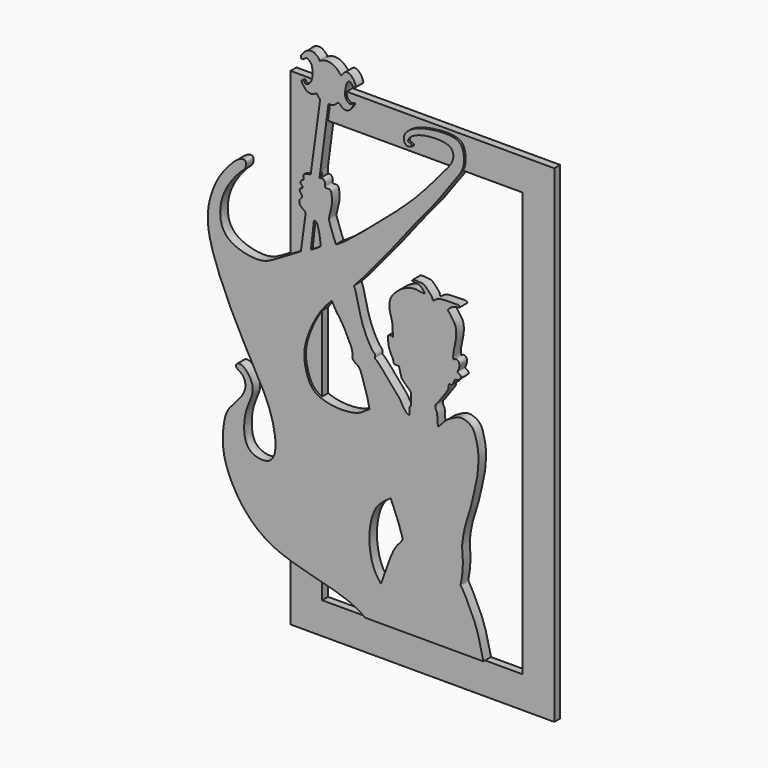
from build123d import *

# Parameters (mm, degrees)
F0_W     = 63.5
F0_H     = 117.348
F0_W_2   = 48.26
F0_H_2   = 102.108
F1_DEPTH = 1.778
F3_DEPTH = 2.286


# Not quite as in the source:
# - the program builds the solid bodies; features that only make, move or delete a surface that nothing else refers to are left out


with BuildPart() as f1:
    # F0 (on Front) → F1 (new body)
    with BuildSketch(Plane.XZ):
        Rectangle(F0_W, F0_H)
        Rectangle(F0_W_2, F0_H_2, mode=Mode.SUBTRACT)
    extrude(amount=F1_DEPTH)

    # F2 (on Front) → F3 (join)
    with BuildSketch(Plane.XZ):
        with BuildLine():
            add(Edge.make_bspline(
                [(-28.8374722004, 21.5742178261), (-30.6445266317, 20.5109243646), (-33.9764528041, 18.5503772709), (-37.8527344031, 16.0868230345), (-43.0809599889, 16.7170062506), (-47.3789384405, 18.794237139), (-48.7167168865, 23.3455521665), (-47.3719498157, 29.1582685078), (-43.3415670037, 33.9108073027), (-42.2121836941, 34.5732882674), (-41.9507977083, 35.938845508), (-42.3333204321, 36.7475829481), (-44.1473400122, 36.3092311493), (-46.6824595583, 33.5416483151), (-49.1001201458, 30.4422843437), (-51.2372465796, 24.8106434738), (-51.4137441027, 19.3675611074), (-49.5817162928, 12.4493998397), (-44.2704702787, 0.3211581031), (-37.1755887329, -11.5642948088), (-35.4487427211, -17.0178211165), (-34.6127773517, -22.0453857416), (-35.8789456032, -25.9302009475), (-40.4306981926, -25.6453855152), (-42.745997505, -22.886153112), (-42.4738766361, -16.7144830815), (-40.6806535744, -13.4910974976), (-40.0664580785, -9.9881086062), (-42.9364872688, -6.6628933305), (-44.5452443837, -7.2761942975), (-44.4760678883, -8.3137831853), (-42.5790186494, -8.9816076925), (-41.7571205036, -12.1114963982), (-44.0992630457, -15.094189727), (-46.4933889074, -17.4101575868), (-47.496752464, -20.5925653051), (-47.9021911924, -26.3457982284), (-46.2453688541, -31.694183229), (-42.9973247437, -37.4039588168), (-36.9486594172, -43.2843741486), (-27.0980961603, -46.0959132992), (-18.253413652, -48.1946158593), (-14.8236518726, -49.9599613249), (-13.3932409808, -51.054)],
                knots=[0, 0, 0, 0, 0.0284685511, 0.0528169742, 0.0787771668, 0.103309748, 0.1270996122, 0.155758436, 0.1840606297, 0.1968852567, 0.2097197675, 0.219193912, 0.2333019746, 0.2556216875, 0.2790051765, 0.3070277116, 0.3336945302, 0.3640754229, 0.4069660437, 0.4502034574, 0.4777618038, 0.503519277, 0.5248205898, 0.5470334855, 0.5680348323, 0.5960679952, 0.6185593645, 0.6397277142, 0.6624220593, 0.6750647171, 0.6847202502, 0.7001335145, 0.7194455011, 0.7415760458, 0.7625548204, 0.783318959, 0.8108258648, 0.8382273683, 0.8676075268, 0.9007486849, 0.9380010364, 0.9729300864, 1, 1, 1, 1], degree=3))
            Line((-13.3932409808, -51.054), (15.1003189385, -51.054))
            add(Edge.make_bspline(
                [(15.1003189385, -51.054), (14.7722900578, -49.5579249437), (14.1020170773, -46.5009420195), (12.7528907462, -42.4071263816), (9.9333743136, -36.9216616198), (9.5084923554, -36.6637727294), (10.1084939934, -34.6288899354), (10.2153280385, -30.3113968011), (9.7980898954, -28.1394697114), (10.7080656026, -23.2601793067), (11.9514711607, -20.1324302445), (13.1010876265, -14.8228655909), (13.7880647157, -11.9419770525), (14.0493109457, -7.5802953221), (13.4511356149, -4.8472904204), (12.76598174, -2.4365194391), (11.1382455413, -1.3567392342), (9.2219650914, -0.9678252802), (7.3083771149, -2.1492742921), (5.8696736679, -2.848096712), (4.1882789673, -5.0959627988), (4.135168267, -4.5844708191), (4.0595196277, -3.9698632766), (3.9494816755, -2.7352020922), (4.0020212061, -1.7641327243), (3.5632580082, -1.4143290493), (3.5736899111, -0.7763326658), (3.540691255, -0.3543819156), (3.7416320683, -0.3021459036), (4.7917091345, 1.1175230461), (6.1100169972, 2.8804211142), (6.517063651, 3.6076468934), (6.7214863109, 4.1127354696), (6.7349267543, 5.0418635371), (6.9661076458, 5.1449629566), (7.2998199393, 4.9472168504), (7.6839640413, 5.2021962898), (7.9465592878, 5.990425857), (8.4411037724, 6.6406894077), (8.6356690767, 6.4645808202), (9.0575243987, 6.5156688466), (9.3471958079, 6.9596361614), (9.6742353766, 7.1529530869), (9.8163270367, 7.5493510729), (9.4282351345, 7.8778861581), (8.9688774098, 8.0999224213), (8.8143574689, 8.2281084507), (9.1513070508, 8.8409313794), (9.4273275691, 9.9365198566), (9.1545649654, 10.6116762274), (8.6157342404, 10.9859416396), (8.0749768769, 10.7027906235), (7.8530908113, 10.5141414795), (7.7709176416, 11.3910350954), (8.0671819779, 13.1379872081), (8.5589206868, 15.1876384685), (8.6107752415, 17.2664258453), (8.0918078208, 18.6782306489), (6.7243838798, 20.4023083098), (6.5180270197, 20.5782720281), (6.8171445504, 21.1002376389), (7.7716875278, 21.7615716184), (9.0146230181, 22.0207510836), (9.2964165831, 21.9736284776), (9.4595139986, 22.3214131369), (9.1489395801, 22.559670012), (8.0009121772, 22.588578332), (6.3568398748, 22.4945920493), (4.1086656354, 22.4417433253), (3.1822703981, 21.5287919381), (2.878260486, 21.4537067759), (2.8163472334, 22.1997911047), (1.8379545777, 23.1596994387), (0.7934880987, 24.2772209795), (0.251112851, 24.2533235367), (-0.5103503454, 24.3619782232), (-1.9562511112, 24.4771290119), (-1.9629547418, 24.1376106862), (-2.2359854926, 23.9849578263), (-1.3327611719, 23.9155363941), (-0.6882391907, 23.8814377374), (0.0870687781, 23.5431004003), (0.8657331386, 22.5941427548), (0.9837039545, 22.3661347589), (0.7252967118, 22.2374071298), (-0.1561133672, 22.3908627429), (-1.7275308646, 22.6688377611), (-4.0003495972, 21.926368016), (-5.6807056374, 20.7391060371), (-7.110076714, 19.1889155011), (-7.5699337902, 17.6279704733), (-7.5479933733, 15.9758608749), (-6.8809655693, 14.0698343391), (-6.7433698114, 12.5692253603), (-6.6983774939, 11.2140473658), (-6.6740917973, 10.4825571179)],
                knots=[0, 0, 0, 0, 0.0213715461, 0.0436692338, 0.0677880785, 0.0737834725, 0.0874759948, 0.1085526933, 0.1240681824, 0.1457298915, 0.1650783154, 0.1880194557, 0.2059184735, 0.2265521967, 0.2436956329, 0.2591264985, 0.2727255483, 0.2863846415, 0.3008650667, 0.3148270791, 0.330027902, 0.3343469628, 0.3424384925, 0.353899676, 0.3635882184, 0.3705812706, 0.3785796712, 0.3847118849, 0.3884234657, 0.4014854067, 0.4170117761, 0.4258507384, 0.4334143682, 0.4428034122, 0.4469952468, 0.4528119876, 0.4589865448, 0.4685076439, 0.4769432216, 0.4811826077, 0.4873164087, 0.4945550584, 0.5007646256, 0.5065813714, 0.5134950894, 0.5207555559, 0.5244912506, 0.5324128735, 0.5432744406, 0.5516195487, 0.5592077583, 0.5668176205, 0.5708917339, 0.5788794197, 0.5926362479, 0.6075307492, 0.6216913688, 0.6345581379, 0.6491130794, 0.6536475225, 0.660564832, 0.6717778203, 0.6829941739, 0.6879304978, 0.693253388, 0.6986683406, 0.7091240408, 0.722497007, 0.7376300971, 0.7485705017, 0.7527623321, 0.7603721885, 0.7725684133, 0.7848030729, 0.7916288884, 0.8008725501, 0.8124036201, 0.817258995, 0.8209946838, 0.8292673352, 0.8379052215, 0.8471668716, 0.8582773827, 0.8625926264, 0.8670078099, 0.8762514714, 0.8890570386, 0.9044362535, 0.9190440561, 0.933434475, 0.9460248741, 0.9588972125, 0.9730515555, 0.9854539223, 1, 1, 1, 1], degree=3))
            add(Edge.make_bspline(
                [(-6.6740917973, 10.4825571179), (-6.7561211567, 10.5936230341), (-6.9356670272, 10.8367241231), (-7.5812960249, 10.8168289248), (-7.9535422563, 10.4978752089), (-7.8334496953, 9.6452525388), (-7.8060153575, 8.4896184547), (-7.4055578058, 7.353658063), (-6.6069295404, 5.9506688631), (-6.5055283788, 4.9687054516), (-6.0061776988, 4.8973217972), (-5.4981649396, 4.9145315299), (-5.3107018852, 4.9127188536), (-5.2330521867, 4.9119680189)],
                knots=[0, 0, 0, 0, 0.0696461782, 0.1524415623, 0.2220877694, 0.3190103741, 0.4363508934, 0.556566394, 0.696357003, 0.7973363862, 0.8667428504, 0.9448031105, 1, 1, 1, 1], degree=3))
            add(Edge.make_bspline(
                [(-5.2330521867, 4.9119680189), (-5.146861191, 4.5660062774), (-4.9682361085, 3.8490236722), (-4.6219056976, 2.5082589892), (-4.2021331969, 2.0962557396), (-2.9657502373, 1.014791874), (-2.5386993366, 0.5490572538), (-2.3540400434, 0.3476708953)],
                knots=[0, 0, 0, 0, 0.2042280102, 0.4232489125, 0.5730933472, 0.8154030804, 1, 1, 1, 1], degree=3))
            add(Edge.make_bspline(
                [(-2.3540400434, 0.3476708953), (-2.3829802065, -0.7602616391), (-2.4212492716, -2.2253377778), (-2.2846284452, -2.6583186613), (-2.5754899011, -2.6518888941), (-2.6576659375, -2.9041605459), (-2.7110750417, -3.5139345271), (-2.6991437306, -4.6763806148), (-2.8608720357, -4.5889391817), (-3.2680155587, -4.5594305596), (-3.7042387415, -4.0478894428), (-4.4818472638, -3.0502813026), (-4.9911704868, -1.8417652687), (-6.2400466725, -0.6681796179), (-7.5159903027, 1.0604646538), (-8.8080861768, 2.4359699083), (-9.7313316767, 3.5304142399), (-10.6258942376, 4.4131900722), (-11.0847683999, 4.7046281777), (-10.9888188166, 4.8231195738), (-10.9759662052, 5.1435101545), (-11.0232788281, 5.6290243907), (-11.4225503118, 5.9120197767), (-12.2163109677, 7.0348670678), (-13.7420414858, 9.8861377176), (-14.797732711, 13.5587762129), (-15.5002809474, 16.938160332), (-15.8927932332, 18.0415119075), (-16.051331535, 18.4871628881)],
                knots=[0, 0, 0, 0, 0.0624316523, 0.0825565829, 0.0993333961, 0.116611376, 0.1486892008, 0.1873856731, 0.198210135, 0.2212164455, 0.2519237926, 0.2946460302, 0.3381120105, 0.3874951872, 0.4437597023, 0.4960942348, 0.542098038, 0.5852791235, 0.6102342892, 0.6219828454, 0.6433253776, 0.669223829, 0.6941932086, 0.737164801, 0.8056426936, 0.8820581998, 0.9523625288, 1, 1, 1, 1], degree=3))
            add(Edge.make_bspline(
                [(-16.051331535, 18.4871628881), (-15.5517599538, 19.002063278), (-14.3074514993, 20.2845519796), (-11.0110254935, 24.4265106413), (-6.3922912305, 29.7509238784), (-2.6663246898, 34.9578645101), (3.7583803847, 42.2838663597), (7.5288904098, 47.9422832888), (10.4603489308, 51.5053514139), (10.5006637912, 54.7850970026), (9.5273500272, 58.1540251755), (2.2062081755, 57.8251890802), (-2.5199613248, 56.3250981069), (-4.451424249, 53.9680622463), (-3.6414750164, 52.0311239105), (-2.5961570773, 52.276186777), (-1.7499666284, 52.5402770499), (-2.3520110164, 53.0602804255), (-3.0923080983, 53.0907935986), (-3.0096197878, 53.9678058697), (-1.3049454768, 55.3708866638), (2.6835566617, 56.1992528071), (7.6172129622, 55.9525743823), (8.2109524433, 52.5899119836), (4.7539736303, 48.7421122955), (-1.1079221789, 41.6228867876), (-9.5330999403, 34.3183933665), (-17.902021111, 27.1755924768), (-19.8029720426, 26.1099277891), (-20.4314477742, 25.7576070726)],
                knots=[0, 0, 0, 0, 0.0291104885, 0.0725069806, 0.1228353295, 0.1713682501, 0.2304070094, 0.2805072828, 0.3198966916, 0.3531340667, 0.3845246828, 0.4333028352, 0.4766252763, 0.507102225, 0.5307607366, 0.5492061783, 0.5642845401, 0.5780946167, 0.5933854864, 0.6077905823, 0.6344342796, 0.6737917328, 0.7135479812, 0.7427729023, 0.784331053, 0.8418574798, 0.9073832371, 0.9693798578, 1, 1, 1, 1], degree=3))
            add(Edge.make_bspline(
                [(-20.4314477742, 25.7576070726), (-21.1502520026, 27.6696138272), (-22.1277741729, 30.2698058108), (-22.0994786833, 30.9199581399), (-21.1024511744, 34.1126049164), (-21.5147228877, 36.6012284558), (-21.8078201152, 36.9648509421), (-22.2530300333, 36.9759859309), (-22.9244144326, 36.9191412282), (-23.0728212936, 37.1463838925), (-22.8924152583, 37.9513815557), (-23.3859868504, 38.6741256382), (-23.8237632485, 38.6709087419), (-24.166001436, 38.6497135982), (-24.3499167264, 38.6383235455)],
                knots=[0, 0, 0, 0, 0.1830315352, 0.2489097538, 0.400063716, 0.5319310397, 0.5809476751, 0.6356504014, 0.7024892313, 0.7392311646, 0.813115092, 0.887151166, 0.9393561945, 1, 1, 1, 1], degree=3))
            add(Edge.make_bspline(
                [(-24.3499167264, 38.6383235455), (-23.6352657278, 44.0906236569), (-22.9206147293, 49.5429237684), (-22.2059637308, 54.9952238798)],
                knots=[0, 0, 0, 0, 16.4968094793, 16.4968094793, 16.4968094793, 16.4968094793], degree=3))
            add(Edge.make_bspline(
                [(-22.2059637308, 54.9952238798), (-21.7124314605, 54.9670072628), (-20.7505167626, 54.9120119154), (-19.8001052819, 56.5231145069), (-18.8369153081, 54.9330769727), (-17.1603288398, 54.8819695725), (-16.2823343308, 56.4961351162), (-16.1707596146, 56.6996835992), (-16.2286252484, 57.0540229256), (-16.7688741771, 56.6450171781), (-17.2823782104, 56.6463035905), (-17.971066275, 57.2856628369), (-18.3271132202, 58.170389398), (-18.0879280294, 59.6871477482), (-17.8354917844, 60.9574221271), (-17.0194534892, 61.5934410664), (-16.4774692094, 60.9448171121), (-16.2941498055, 60.3767668537), (-15.6893658989, 60.4500229567), (-15.5653924714, 61.0448732044), (-16.2888798172, 62.3905210002), (-17.3879567263, 63.3021914263), (-18.4223353732, 63.0380493941), (-19.0313931536, 61.9504219929), (-19.2872479384, 62.089093047), (-20.0180961772, 63.0787371036), (-21.5075939979, 63.9846226985), (-23.4556140785, 64.0057651604), (-24.451171157, 63.2665261649), (-24.2345410492, 63.6493698771), (-25.2350050779, 64.5031908369), (-25.930081291, 64.9278961485), (-27.3221915669, 64.8166341037), (-28.4816176113, 63.6719357686), (-28.9912554415, 62.8829267507), (-28.7372631395, 62.4034521887), (-28.3976670379, 62.3932650764), (-27.8507960215, 62.701807995), (-27.4325876343, 63.2090601189), (-26.1000186041, 62.0783156798), (-26.0827457192, 60.6405803597), (-26.0162238853, 59.0783763065), (-26.6086994649, 57.9684083004), (-27.2514142293, 57.3902348887), (-28.0214530918, 57.5227821286), (-28.1179679209, 58.2155216822), (-28.9178798033, 57.7746688393), (-28.2459160737, 56.9178392), (-27.5010410377, 55.843977488), (-25.9304672609, 55.6005301831), (-25.2623234404, 56.2667150344), (-24.9730728155, 56.2882859884), (-24.7190570268, 55.7267041268), (-24.3312567555, 55.401429237), (-24.2818922766, 55.249848659), (-24.2133978754, 55.2072972059)],
                knots=[0, 0, 0, 0, 0.0242703586, 0.0474355849, 0.070902422, 0.0955823308, 0.1218530765, 0.1319634207, 0.141091261, 0.1559220404, 0.1703915436, 0.189369363, 0.2091040349, 0.2343381435, 0.257962604, 0.2759492794, 0.2929235986, 0.3081648115, 0.3215943411, 0.3356411548, 0.3608226731, 0.3846613019, 0.4046036003, 0.4260062989, 0.4342648989, 0.4561381452, 0.4835265843, 0.5124689126, 0.5314647786, 0.539576457, 0.5620677979, 0.5812820074, 0.6042025786, 0.6304283001, 0.6495035665, 0.6625915151, 0.673556673, 0.6896722935, 0.7042150976, 0.7284209008, 0.7532383145, 0.7786693531, 0.801275186, 0.8196431416, 0.8358938646, 0.8502407707, 0.8648842801, 0.8840376642, 0.9078962127, 0.9323430654, 0.9511564773, 0.9603078201, 0.9758196834, 0.9904617098, 1, 1, 1, 1], degree=3))
            add(Edge.make_bspline(
                [(-26.4855902642, 38.6383235455), (-25.692521284, 44.1613147656), (-25.0064668556, 49.6843059858), (-24.2133978754, 55.2072972059)],
                knots=[0, 0, 0, 0, 16.7240469508, 16.7240469508, 16.7240469508, 16.7240469508], degree=3))
            add(Edge.make_bspline(
                [(-26.4855902642, 38.6383235455), (-26.9603676474, 38.5468430051), (-27.7398169437, 38.3966580018), (-28.3215093002, 38.042787906), (-28.1268681612, 37.4376150555), (-28.1642454173, 37.0395994683), (-28.3334211593, 36.772003224), (-28.7781304879, 36.7376075304), (-29.1090098129, 35.9193703303), (-28.3136983855, 35.5123947072), (-28.4462692408, 34.990083717), (-29.3318464541, 34.8030972168), (-28.9338380092, 33.8851528263), (-28.4157002113, 33.3801439281), (-28.7068542961, 32.9267695538), (-29.2774617195, 32.4160468652), (-29.2716396945, 31.3411322002), (-28.273247251, 30.6628525547), (-27.8657508194, 30.3340969404), (-27.6827570051, 30.1864631474)],
                knots=[0, 0, 0, 0, 0.0842343611, 0.1382888398, 0.1926204681, 0.2389472394, 0.2769293335, 0.3230421014, 0.3830717542, 0.4456721286, 0.490554076, 0.5514070634, 0.6164245541, 0.6766884483, 0.7243812954, 0.7875286204, 0.8578701541, 0.9361739623, 1, 1, 1, 1], degree=3))
            add(Edge.make_bspline(
                [(-27.6827570051, 30.1864631474), (-28.0676620702, 27.315714707), (-28.4525671353, 24.4449662666), (-28.8374722004, 21.5742178261)],
                knots=[0, 0, 0, 0, 8.689311633, 8.689311633, 8.689311633, 8.689311633], degree=3))
        make_face()
        with BuildLine():
            add(Edge.make_bspline(
                [(-21.3782601058, 13.5360965505), (-22.049780904, 12.8760856138), (-23.5734598364, 11.3785225268), (-26.0689817022, 7.3142632198), (-28.0241678252, 2.234909865), (-28.1633571843, -1.7337546998), (-26.6198497273, -6.7715449647), (-23.5162984383, -8.2696864364), (-19.5697539261, -9.0442761398), (-14.83914754, -8.4586717071), (-13.298398895, -7.0373091229), (-12.6053780197, -6.708897943), (-12.3156383634, -6.5715950914)],
                knots=[0, 0, 0, 0, 0.0916388663, 0.2079283476, 0.3312117296, 0.4380575861, 0.5553442883, 0.6498260432, 0.7574114207, 0.872094786, 0.9465251134, 1, 1, 1, 1], degree=3))
            add(Edge.make_bspline(
                [(-12.3156383634, -6.5715950914), (-12.483275002, -5.7062855342), (-12.8419708272, -3.8547635264), (-14.0216733084, -0.4952418499), (-14.6365865126, 1.6515265591), (-16.0842787597, 2.333083491), (-16.5146541062, 2.9346022679), (-16.2576440001, 4.3053399889), (-17.4722742272, 6.9928122818), (-19.1816731709, 10.1628320053), (-20.4101560735, 11.6009952084), (-21.0493756913, 12.8787036974), (-21.3782601058, 13.5360965505)],
                knots=[0, 0, 0, 0, 0.1141513568, 0.2442521841, 0.3452170126, 0.4270308061, 0.4814834939, 0.5569605145, 0.6752574605, 0.8062607377, 0.9003193549, 1, 1, 1, 1], degree=3))
        make_face(mode=Mode.SUBTRACT)
        with BuildLine():
            add(Edge.make_bspline(
                [(-7.2220843285, -23.7149521708), (-8.4094839327, -24.5312578811), (-10.7973795769, -26.1728727536), (-12.2302933578, -30.5104025543), (-12.5480537993, -35.0905666599), (-11.5199854756, -40.102294166), (-10.1657159735, -41.8723247418), (-9.5679583028, -42.653594166)],
                knots=[0, 0, 0, 0, 0.1995314422, 0.4012636185, 0.6118457457, 0.8286735524, 1, 1, 1, 1], degree=3))
            add(Edge.make_bspline(
                [(-7.2220843285, -23.7149521708), (-6.7191271422, -24.8817049803), (-5.7229867482, -27.1925370651), (-4.3482367915, -31.0235311576), (-4.3475486625, -31.8649081506), (-6.3823353868, -33.6318707888), (-8.0463630827, -38.385472654), (-9.0696849801, -41.2559221313), (-9.5679583028, -42.653594166)],
                knots=[0, 0, 0, 0, 0.186636248, 0.3696455894, 0.4468424256, 0.589688755, 0.8002122813, 1, 1, 1, 1], degree=3))
        make_face(mode=Mode.SUBTRACT)
        with BuildLine():
            add(Edge.make_bspline(
                [(-25.7101207972, 29.1279740632), (-25.9506863852, 26.978922387), (-26.1912519733, 24.8298707108), (-26.4318175614, 22.6808190346)],
                knots=[0, 0, 0, 0, 6.4874227689, 6.4874227689, 6.4874227689, 6.4874227689], degree=3))
            add(Edge.make_bspline(
                [(-26.4318175614, 22.6808190346), (-25.8263771847, 22.9751601946), (-25.0714254236, 23.5359142487), (-24.3747535822, 23.8682677707), (-24.0160707605, 24.2610159876), (-24.1249021997, 24.4151656861), (-24.1736086869, 25.8150917995), (-24.5789073995, 27.6877607062), (-25.026760174, 29.0924808163), (-25.5064067139, 29.1162201012), (-25.7101207972, 29.1279740632)],
                knots=[0, 0, 0, 0, 0.1676481449, 0.2818766967, 0.3676604467, 0.4151206269, 0.5623562329, 0.7532180947, 0.9017689508, 1, 1, 1, 1], degree=3))
        make_face(mode=Mode.SUBTRACT)
    extrude(amount=F3_DEPTH)


solid = f1.part
